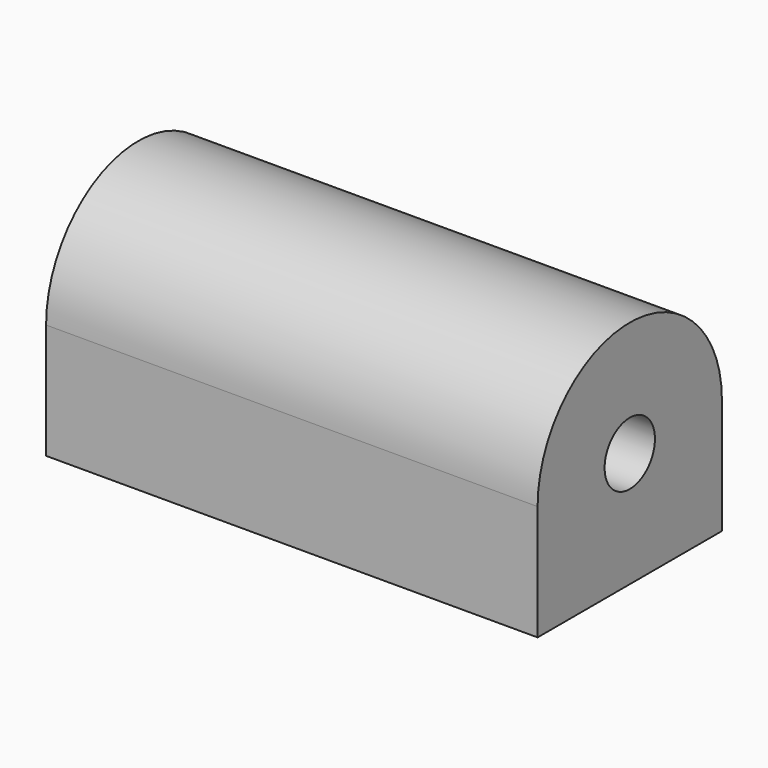
from build123d import *

# Parameters (mm, degrees)
F0_R     = 1.6256
F1_DEPTH = 12.7
F3_DEPTH = 1.27
F2_R     = 1.5875
F4_DEPTH = 1.27
F5_DEPTH = 12.7


# Not quite as in the source:
# - a feature names something its author has since deleted; it is built from what else it names


with BuildPart() as f1:
    # F0 (on Right) → F1 (new body)
    with BuildSketch(Plane.YZ):
        with BuildLine():
            ThreePointArc((0, -5.953125), (4.2094950568, -4.2094950568), (5.953125, 0))
            ThreePointArc((5.953125, 0), (0, 5.953125), (-5.953125, 0))
            ThreePointArc((-5.953125, 0), (-4.2094950568, -4.2094950568), (0, -5.953125))
        make_face()
        Circle(F0_R, mode=Mode.SUBTRACT)
        with BuildLine():
            Line((5.953125, -5.953125), (5.953125, 0))
            ThreePointArc((5.953125, 0), (4.2094950568, -4.2094950568), (0, -5.953125))
            Line((0, -5.953125), (5.953125, -5.953125))
        make_face()
        with BuildLine():
            ThreePointArc((0, -5.953125), (-4.2094950568, -4.2094950568), (-5.953125, 0))
            Line((-5.953125, 0), (-5.953125, -5.953125))
            Line((-5.953125, -5.953125), (0, -5.953125))
        make_face()
    extrude(amount=F1_DEPTH)

    # F0 (on Right) → F5 (join)
    with BuildSketch(Plane.YZ):
        with BuildLine():
            ThreePointArc((0, -5.953125), (4.2094950568, -4.2094950568), (5.953125, 0))
            ThreePointArc((5.953125, 0), (0, 5.953125), (-5.953125, 0))
            ThreePointArc((-5.953125, 0), (-4.2094950568, -4.2094950568), (0, -5.953125))
        make_face()
        Circle(F0_R, mode=Mode.SUBTRACT)
        with BuildLine():
            Line((5.953125, -5.953125), (5.953125, 0))
            ThreePointArc((5.953125, 0), (4.2094950568, -4.2094950568), (0, -5.953125))
            Line((0, -5.953125), (5.953125, -5.953125))
        make_face()
        with BuildLine():
            ThreePointArc((0, -5.953125), (-4.2094950568, -4.2094950568), (-5.953125, 0))
            Line((-5.953125, 0), (-5.953125, -5.953125))
            Line((-5.953125, -5.953125), (0, -5.953125))
        make_face()
    extrude(amount=-F5_DEPTH)


with BuildPart() as f3:
    # F0 (on Right) → F3 (new body)
    with BuildSketch(Plane.YZ):
        Circle(F0_R)
    extrude(amount=F3_DEPTH)


with BuildPart() as f4:
    # F2 (on Right) → F4 (new body)
    with BuildSketch(Plane.YZ):
        Circle(F2_R)
    extrude(amount=-F4_DEPTH)


solid = Compound([f1.part, f3.part, f4.part])
